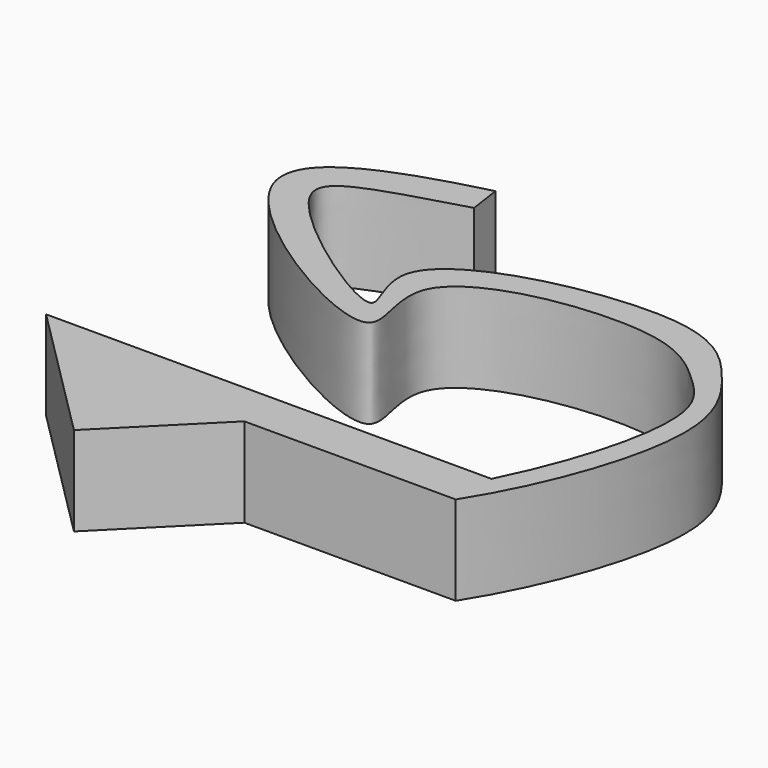
from build123d import *

# Parameters (mm, degrees)
F1_DEPTH = 10


with BuildPart() as f1:
    # F0 (on Top) → F1 (new body)
    with BuildSketch(Plane.XY):
        with BuildLine():
            add(Edge.make_bspline(
                [(65.6013534163, 30.2538078813), (69.289300658, 37.6297165635), (72.920266298, 50.710224191), (67.1358590378, 56.3463392384), (60.1349727263, 62.4430867521), (33.3157509535, 58.2679344594), (44.7870704091, 39.9864018122), (6.3423304614, 62.3170224179), (18.8733997605, 69.8270832108), (31.8217124655, 73.0483756965)],
                knots=[0, 0, 0, 0, 0.1688825653, 0.2622409242, 0.3751546432, 0.5437640281, 0.6473760323, 0.8364637952, 1, 1, 1, 1], degree=3))
            Line((65.6013534163, 30.2538078813), (15.6985400292, 30.2538078813))
            Line((15.6985400292, 30.2538078813), (31.305141747, 14.6472061635))
            Line((31.305141747, 14.6472061635), (41.9117434648, 25.2538078813))
            Line((41.9117434648, 25.2538078813), (65.6013534163, 25.2538078813))
            add(Edge.make_bspline(
                [(65.6013534163, 25.2538078813), (70.1094575825, 32.337968029), (76.0142255488, 48.6856865488), (69.1296123169, 58.6003414204), (61.1289969269, 66.5277757677), (29.8172914541, 59.8483736861), (41.835650349, 44.3564532244), (13.0411962613, 64.0377724232), (21.4317883919, 66.2436371114), (32.3480498046, 69.3968422711)],
                knots=[0, 0, 0, 0, 0.181690496, 0.2994927091, 0.4211723284, 0.6036374989, 0.6965292525, 0.8607043342, 1, 1, 1, 1], degree=3))
            Line((32.3480498046, 69.3968422711), (31.8217124655, 73.0483756965))
        make_face()
    extrude(amount=F1_DEPTH)


solid = f1.part
